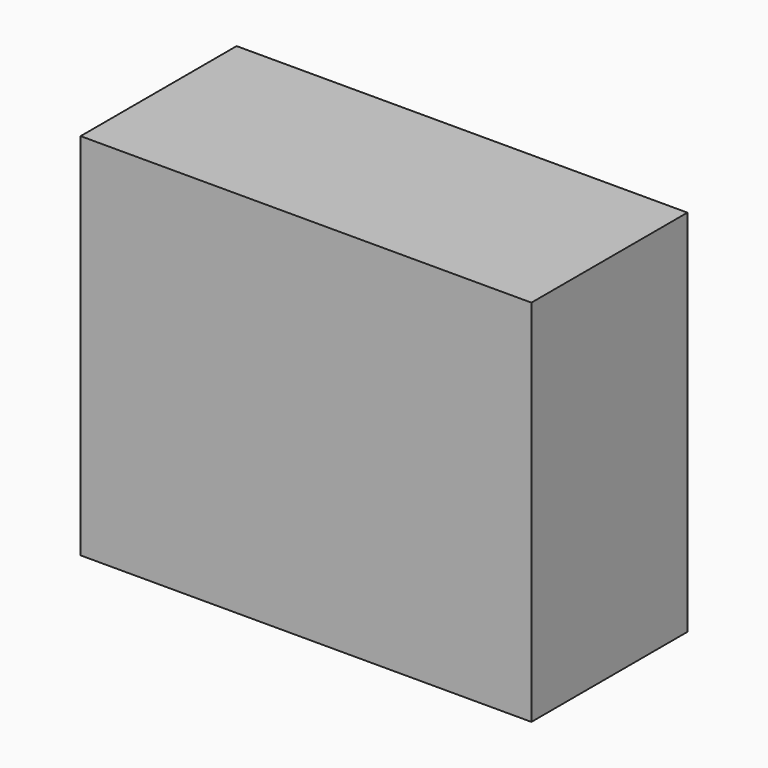
from build123d import *

# Parameters (mm, degrees)
F0_W     = 58.7265528738
F0_H     = 48.0848290026
F1_DEPTH = 25.4
F2_R     = 10.0505175069
F3_DEPTH = 25.4


# Not quite as in the source:
# - the program builds the solid bodies; features that only make, move or delete a surface that nothing else refers to are left out


with BuildPart() as f1:
    # F0 (on Front) → F1 (new body)
    with BuildSketch(Plane.XZ):
        with Locations((2.5618970394, 0)):
            Rectangle(F0_W, F0_H)
    extrude(amount=F1_DEPTH)

    # F2 (on Front) → F3 (join)
    with BuildSketch(Plane.XZ):
        Circle(F2_R)
    extrude(amount=F3_DEPTH)


solid = f1.part
